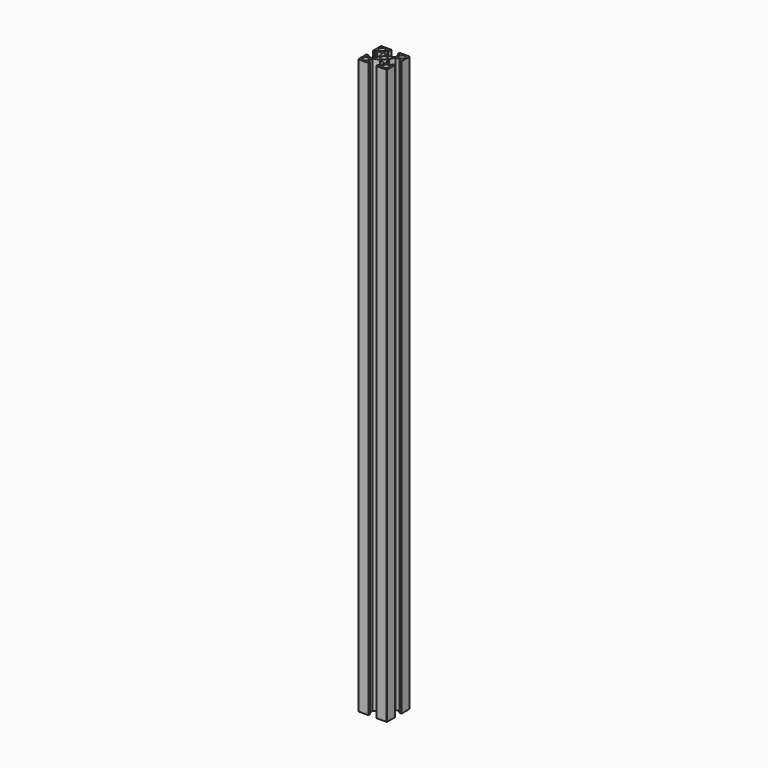
from build123d import *

# Parameters (mm, degrees)
F1_DEPTH = 400


# Not quite as in the source:
# - ends of sketch curves that miss each other by under 0.0002 mm in the source are joined


with BuildPart() as f1:
    # F0 (on Top) → F1 (new body)
    with BuildSketch(Plane.XY):
        with BuildLine():
            ThreePointArc((0, 2.15), (1.5202795796, 1.5202795796), (2.15, 0))
            Line((2.15, 0), (3, 0))
            Line((3, 0), (3.307278, 0.307278))
            ThreePointArc((3.307278, 0.307278), (3.7143803747, 2.2820219924), (4.7078187099, 4.0365664363))
            ThreePointArc((4.7078187099, 4.0365664363), (4.812308461, 4.1201573706), (4.94275, 4.15))
            Line((4.94275, 4.15), (8.2, 4.15))
            ThreePointArc((8.2, 4.15), (8.4121320344, 4.0621320344), (8.5, 3.85))
            Line((8.5, 3.85), (8.5, 2.95))
            ThreePointArc((8.5, 2.95), (8.5878679656, 2.7378679656), (8.8, 2.65))
            Line((8.8, 2.65), (9.7, 2.65))
            ThreePointArc((9.7, 2.65), (9.9121320344, 2.7378679656), (10, 2.95))
            Line((10, 2.95), (10, 9.7))
            ThreePointArc((10, 9.7), (9.9121320344, 9.9121320344), (9.7, 10))
            Line((9.7, 10), (2.95, 10))
            ThreePointArc((2.95, 10), (2.7378679656, 9.9121320344), (2.65, 9.7))
            Line((2.65, 9.7), (2.65, 8.8))
            ThreePointArc((2.65, 8.8), (2.7378679656, 8.5878679656), (2.95, 8.5))
            Line((2.95, 8.5), (3.85, 8.5))
            ThreePointArc((3.85, 8.5), (4.0621320344, 8.4121320344), (4.15, 8.2))
            Line((4.15, 8.2), (4.15, 4.94275))
            ThreePointArc((4.15, 4.94275), (4.1201572004, 4.8123081084), (4.036566086, 4.7078178916))
            ThreePointArc((4.036566086, 4.7078178916), (2.2820216259, 3.7143802371), (0.3072779813, 3.3072783955))
            Line((0.3072779813, 3.3072783955), (0, 3))
            Line((0, 3), (0, 2.15))
        make_face()
        with BuildLine():
            ThreePointArc((7, 9), (8.4142135624, 8.4142135624), (9, 7))
            ThreePointArc((9, 7), (8.4142135624, 5.5857864376), (7, 5))
            ThreePointArc((7, 5), (5.5857864376, 5.5857864376), (5, 7))
            ThreePointArc((5, 7), (5.5857864376, 8.4142135624), (7, 9))
        make_face(mode=Mode.SUBTRACT)
        with BuildLine():
            Line((3, 0), (2.15, 0))
            ThreePointArc((2.15, 0), (1.5202795796, -1.5202795796), (0, -2.15))
            Line((0, -2.15), (0, -3))
            Line((0, -3), (0.307278, -3.307277))
            ThreePointArc((0.307278, -3.307277), (2.2820216259, -3.7143792371), (4.036565823, -4.7078172229))
            ThreePointArc((4.036565823, -4.7078172229), (4.1201572004, -4.8123071084), (4.15, -4.942749))
            Line((4.15, -4.942749), (4.15, -8.2))
            ThreePointArc((4.15, -8.2), (4.0621320344, -8.4121320344), (3.85, -8.5))
            Line((3.85, -8.5), (2.95, -8.5))
            ThreePointArc((2.95, -8.5), (2.7378679656, -8.5878679656), (2.65, -8.8))
            Line((2.65, -8.8), (2.65, -9.7))
            ThreePointArc((2.65, -9.7), (2.7378679656, -9.9121320344), (2.95, -10))
            Line((2.95, -10), (9.7, -10))
            ThreePointArc((9.7, -10), (9.9121320344, -9.9121320344), (10, -9.7))
            Line((10, -9.7), (10, -2.95))
            ThreePointArc((10, -2.95), (9.9121320344, -2.7378679656), (9.7, -2.65))
            Line((9.7, -2.65), (8.8, -2.65))
            ThreePointArc((8.8, -2.65), (8.5878679656, -2.7378679656), (8.5, -2.95))
            Line((8.5, -2.95), (8.5, -3.85))
            ThreePointArc((8.5, -3.85), (8.4121320344, -4.0621320344), (8.2, -4.15))
            Line((8.2, -4.15), (4.94275, -4.15))
            ThreePointArc((4.94275, -4.15), (4.8123081084, -4.1201572004), (4.7078178916, -4.036566086))
            ThreePointArc((4.7078178916, -4.036566086), (3.7143800615, -2.2820211583), (3.3072783483, -0.3072769835))
            Line((3.3072783483, -0.3072769835), (3, 0))
        make_face()
        with BuildLine():
            ThreePointArc((7, -5), (8.4142135624, -5.5857864376), (9, -7))
            ThreePointArc((9, -7), (8.4142135624, -8.4142135624), (7, -9))
            ThreePointArc((7, -9), (5.5857864376, -8.4142135624), (5, -7))
            ThreePointArc((5, -7), (5.5857864376, -5.5857864376), (7, -5))
        make_face(mode=Mode.SUBTRACT)
        with BuildLine():
            Line((0, -3), (0, -2.15))
            ThreePointArc((0, -2.15), (-1.5202795796, -1.5202795796), (-2.15, 0))
            Line((-2.15, 0), (-3, 0))
            Line((-3, 0), (-3.307277, -0.307277))
            ThreePointArc((-3.307277, -0.307277), (-3.7143790615, -2.2820211583), (-4.7078172229, -4.036565823))
            ThreePointArc((-4.7078172229, -4.036565823), (-4.8123071084, -4.1201572004), (-4.942749, -4.15))
            Line((-4.942749, -4.15), (-8.2, -4.15))
            ThreePointArc((-8.2, -4.15), (-8.4121320344, -4.0621320344), (-8.5, -3.85))
            Line((-8.5, -3.85), (-8.5, -2.95))
            ThreePointArc((-8.5, -2.95), (-8.5878679656, -2.7378679656), (-8.8, -2.65))
            Line((-8.8, -2.65), (-9.7, -2.65))
            ThreePointArc((-9.7, -2.65), (-9.9121320344, -2.7378679656), (-10, -2.95))
            Line((-10, -2.95), (-10, -9.7))
            ThreePointArc((-10, -9.7), (-9.9121320344, -9.9121320344), (-9.7, -10))
            Line((-9.7, -10), (-2.95, -10))
            ThreePointArc((-2.95, -10), (-2.7378679656, -9.9121320344), (-2.65, -9.7))
            Line((-2.65, -9.7), (-2.65, -8.8))
            ThreePointArc((-2.65, -8.8), (-2.7378679656, -8.5878679656), (-2.95, -8.5))
            Line((-2.95, -8.5), (-3.85, -8.5))
            ThreePointArc((-3.85, -8.5), (-4.0621320344, -8.4121320344), (-4.15, -8.2))
            Line((-4.15, -8.2), (-4.15, -4.942749))
            ThreePointArc((-4.15, -4.942749), (-4.1201572004, -4.8123071084), (-4.036566086, -4.7078168916))
            ThreePointArc((-4.036566086, -4.7078168916), (-2.2820211583, -3.7143790615), (-0.3072769835, -3.3072773483))
            Line((-0.3072769835, -3.3072773483), (0, -3))
        make_face()
        with BuildLine():
            ThreePointArc((-7, -9), (-8.4142135624, -8.4142135624), (-9, -7))
            ThreePointArc((-9, -7), (-8.4142135624, -5.5857864376), (-7, -5))
            ThreePointArc((-7, -5), (-5.5857864376, -5.5857864376), (-5, -7))
            ThreePointArc((-5, -7), (-5.5857864376, -8.4142135624), (-7, -9))
        make_face(mode=Mode.SUBTRACT)
        with BuildLine():
            ThreePointArc((-2.15, 0), (-1.5202795796, 1.5202795796), (0, 2.15))
            Line((0, 2.15), (0, 3))
            Line((0, 3), (-0.307277, 3.307278))
            ThreePointArc((-0.307277, 3.307278), (-2.2820211583, 3.7143800615), (-4.036565823, 4.7078182229))
            ThreePointArc((-4.036565823, 4.7078182229), (-4.1201572004, 4.8123081084), (-4.15, 4.94275))
            Line((-4.15, 4.94275), (-4.15, 8.2))
            ThreePointArc((-4.15, 8.2), (-4.0621320344, 8.4121320344), (-3.85, 8.5))
            Line((-3.85, 8.5), (-2.95, 8.5))
            ThreePointArc((-2.95, 8.5), (-2.7378679656, 8.5878679656), (-2.65, 8.8))
            Line((-2.65, 8.8), (-2.65, 9.7))
            ThreePointArc((-2.65, 9.7), (-2.7378679656, 9.9121320344), (-2.95, 10))
            Line((-2.95, 10), (-9.7, 10))
            ThreePointArc((-9.7, 10), (-9.9121320344, 9.9121320344), (-10, 9.7))
            Line((-10, 9.7), (-10, 2.95))
            ThreePointArc((-10, 2.95), (-9.9121320344, 2.7378679656), (-9.7, 2.65))
            Line((-9.7, 2.65), (-8.8, 2.65))
            ThreePointArc((-8.8, 2.65), (-8.5878679656, 2.7378679656), (-8.5, 2.95))
            Line((-8.5, 2.95), (-8.5, 3.85))
            ThreePointArc((-8.5, 3.85), (-8.4121320344, 4.0621320344), (-8.2, 4.15))
            Line((-8.2, 4.15), (-4.942749, 4.15))
            ThreePointArc((-4.942749, 4.15), (-4.812307461, 4.1201573706), (-4.7078173786, 4.0365666993))
            ThreePointArc((-4.7078173786, 4.0365666993), (-3.7143793747, 2.2820219924), (-3.3072773955, 0.3072779813))
            Line((-3.3072773955, 0.3072779813), (-3, 0))
            Line((-3, 0), (-2.15, 0))
        make_face()
        with BuildLine():
            ThreePointArc((-7, 5), (-8.4142135624, 5.5857864376), (-9, 7))
            ThreePointArc((-9, 7), (-8.4142135624, 8.4142135624), (-7, 9))
            ThreePointArc((-7, 9), (-5.5857864376, 8.4142135624), (-5, 7))
            ThreePointArc((-5, 7), (-5.5857864376, 5.5857864376), (-7, 5))
        make_face(mode=Mode.SUBTRACT)
    extrude(amount=F1_DEPTH)


solid = f1.part
